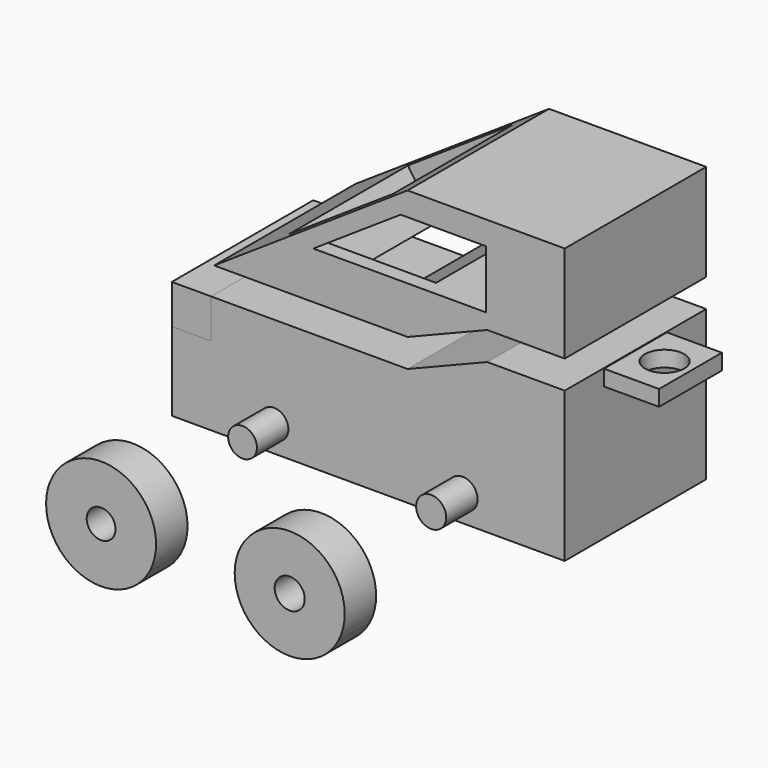
from build123d import *

# Parameters (mm, degrees)
F1_DEPTH       = 57.15
F0_R           = 4.6528750416
F0_R_2         = 4.8589048732
F0_W           = 12.7
F0_H           = 12.7
F2_DEPTH       = 57.15
F3_DEPTH       = 57.15
F4_DEPTH       = 12.7
F6_W           = 40.64
F6_H           = 48.26
F7_DEPTH       = 25.4
F8_W           = 25.4
F8_H           = 5.08
F9_DEPTH       = 17.78
F10_R          = 6.35
F11_DEPTH      = 25.4
F12_R          = 4.6528736
F13_DEPTH      = 82.55
F14_DEPTH      = 69.85
F14_DEPTH_BACK = 12.7


# Not quite as in the source:
# - a feature names something its author has since deleted; it is built from what else it names


with BuildPart() as f1:
    # F0 (on Front) → F1 (new body)
    with BuildSketch(Plane.XZ):
        Polygon((64.6229624206, 40.4410248846), (13.8229624206, 40.4410248846), (-48.6991375794, -1.2403751154), (13.8229624206, -1.2403751154), (39.5902469754, 9.1186), (64.6229624206, 9.1186), align=None)
        Polygon((39.2229624206, 32.8210248846), (39.2229624206, 13.9996248846), (-16.6570375794, 13.9996248846), (11.5750624206, 32.8210248846), align=None, mode=Mode.SUBTRACT)
    extrude(amount=F1_DEPTH)

    # F6 (on face) → F7 (cut)
    with BuildSketch(Plane(origin=(-14.4118692019, 0, 21.6178038029), x_dir=(0.8320502943, 0, 0.5547001962), z_dir=(-0.5547001962, 0, 0.8320502943))):
        with Locations((3.4540443897, -28.3083)):
            Rectangle(F6_W, F6_H)
    extrude(amount=-F7_DEPTH, mode=Mode.SUBTRACT)


with BuildPart() as f1b:
    # F0 (on Front) → F1, piece 2 (new body)
    with BuildSketch(Plane.XZ):
        with BuildLine():
            Line((64.6229624206, -48.4589751154), (64.6229624206, 0))
            Line((64.6229624206, 0), (39.5902469754, 0))
            Line((39.5902469754, 0), (13.8229624206, -10.3589751154))
            Line((13.8229624206, -10.3589751154), (-49.6770375794, -10.3589751154))
            Line((-49.6770375794, -10.3589751154), (-49.6770375794, -23.0589751154))
            Line((-49.6770375794, -23.0589751154), (-62.3770375794, -23.0589751154))
            Line((-62.3770375794, -23.0589751154), (-62.3770375794, -48.4589751154))
            Line((-62.3770375794, -48.4589751154), (-45.0372951028, -48.4589751154))
            ThreePointArc((-45.0372951028, -48.4589751154), (-33.6775364646, -22.8298974098), (-11.5770375794, -40.0769751154))
            ThreePointArc((-11.5770375794, -40.0769751154), (-12.1099598738, -44.3974740006), (-13.676780056, -48.4589751154))
            Line((-13.676780056, -48.4589751154), (15.9227048972, -48.4589751154))
            ThreePointArc((15.9227048972, -48.4589751154), (27.2824635354, -22.8298974098), (49.3829624206, -40.0769751154))
            ThreePointArc((49.3829624206, -40.0769751154), (48.8500401262, -44.3974740006), (47.283219944, -48.4589751154))
            Line((47.283219944, -48.4589751154), (64.6229624206, -48.4589751154))
        make_face()
        with BuildLine():
            ThreePointArc((-11.5770375794, -40.0769751154), (-33.6775364646, -22.8298974098), (-45.0372951028, -48.4589751154))
            Line((-45.0372951028, -48.4589751154), (-13.676780056, -48.4589751154))
            ThreePointArc((-13.676780056, -48.4589751154), (-12.1099598738, -44.3974740006), (-11.5770375794, -40.0769751154))
        make_face()
        with Locations((-29.3570375794, -40.0769751154)):
            Circle(F0_R, mode=Mode.SUBTRACT)
        with BuildLine():
            Line((15.9227048972, -48.4589751154), (47.283219944, -48.4589751154))
            ThreePointArc((47.283219944, -48.4589751154), (48.8500401262, -44.3974740006), (49.3829624206, -40.0769751154))
            ThreePointArc((49.3829624206, -40.0769751154), (27.2824635354, -22.8298974098), (15.9227048972, -48.4589751154))
        make_face()
        with Locations((31.6029624206, -40.0769751154)):
            Circle(F0_R_2, mode=Mode.SUBTRACT)
    extrude(amount=F1_DEPTH)

    # F8 (on face) → F9 (join)
    with BuildSketch(Plane.YZ.offset(64.6229624206)):
        with Locations((-28.575, -2.7389751154)):
            Rectangle(F8_W, F8_H)
    extrude(amount=F9_DEPTH)

    # F10 (on face) → F11 (cut)
    with BuildSketch(Plane.XY.offset(-0.1989751154)):
        with Locations((74.0482390532, -28.5862853714)):
            Circle(F10_R)
    extrude(amount=-F11_DEPTH, mode=Mode.SUBTRACT)


with BuildPart() as f2:
    # F0 (on Front) → F2 (new body)
    with BuildSketch(Plane.XZ):
        with Locations((-56.0270375794, -16.7089751154)):
            Rectangle(F0_W, F0_H)
    extrude(amount=F2_DEPTH)


with BuildPart() as f3:
    # F0 (on Front) → F3 (new body)
    with BuildSketch(Plane.XZ):
        with Locations((-56.0270375794, -16.7089751154)):
            Rectangle(F0_W, F0_H)
    extrude(amount=F3_DEPTH)


with BuildPart() as f4:
    # F0 (on Front) → F4 (new body)
    with BuildSketch(Plane.XZ):
        with BuildLine():
            ThreePointArc((-11.5770375794, -40.0769751154), (-33.6775364646, -22.8298974098), (-45.0372951028, -48.4589751154))
            Line((-45.0372951028, -48.4589751154), (-13.676780056, -48.4589751154))
            ThreePointArc((-13.676780056, -48.4589751154), (-12.1099598738, -44.3974740006), (-11.5770375794, -40.0769751154))
        make_face()
        with Locations((-29.3570375794, -40.0769751154)):
            Circle(F0_R, mode=Mode.SUBTRACT)
        with BuildLine():
            Line((-13.676780056, -48.4589751154), (-45.0372951028, -48.4589751154))
            ThreePointArc((-45.0372951028, -48.4589751154), (-29.3570375794, -57.8569751154), (-13.676780056, -48.4589751154))
        make_face()
    extrude(amount=-F4_DEPTH)


with BuildPart() as f4b:
    # F0 (on Front) → F4, piece 2 (new body)
    with BuildSketch(Plane.XZ):
        with BuildLine():
            Line((15.9227048972, -48.4589751154), (47.283219944, -48.4589751154))
            ThreePointArc((47.283219944, -48.4589751154), (48.8500401262, -44.3974740006), (49.3829624206, -40.0769751154))
            ThreePointArc((49.3829624206, -40.0769751154), (27.2824635354, -22.8298974098), (15.9227048972, -48.4589751154))
        make_face()
        with Locations((31.6029624206, -40.0769751154)):
            Circle(F0_R_2, mode=Mode.SUBTRACT)
        with BuildLine():
            ThreePointArc((15.9227048972, -48.4589751154), (31.6029624206, -57.8569751154), (47.283219944, -48.4589751154))
            Line((47.283219944, -48.4589751154), (15.9227048972, -48.4589751154))
        make_face()
    extrude(amount=-F4_DEPTH)


with BuildPart() as f5_1:
    # F5: instance of F4b
    add(f4b.part.mirror(Plane(origin=(6.4473087682, -57.15, -27.6324476471), x_dir=(1, 0, 0), z_dir=(0, -1, 0))))


with BuildPart() as f5_2:
    # F5: instance of F4
    add(f4.part.mirror(Plane(origin=(6.4473087682, -57.15, -27.6324476471), x_dir=(1, 0, 0), z_dir=(0, -1, 0))))


with BuildPart() as f13:
    # F12 (on face) → F13 (new body)
    with BuildSketch(Plane(origin=(0, 12.7, 0), x_dir=(-1, 0, 0), z_dir=(0, 1, 0))):
        with Locations((29.3570375794, -40.0769751154)):
            Circle(F12_R)
    extrude(amount=-F13_DEPTH)


with BuildPart() as f14:
    # F0 (on Front) → F14 (new body, two sides)
    with BuildSketch(Plane.XZ) as f14_sk:
        with Locations((31.6029624206, -40.0769751154)):
            Circle(F0_R_2)
    extrude(amount=F14_DEPTH)
    extrude(f14_sk.sketch, amount=-F14_DEPTH_BACK)


solid = Compound([f1.part, f1b.part, f2.part, f3.part, f4.part, f4b.part, f5_1.part, f5_2.part, f13.part, f14.part])
